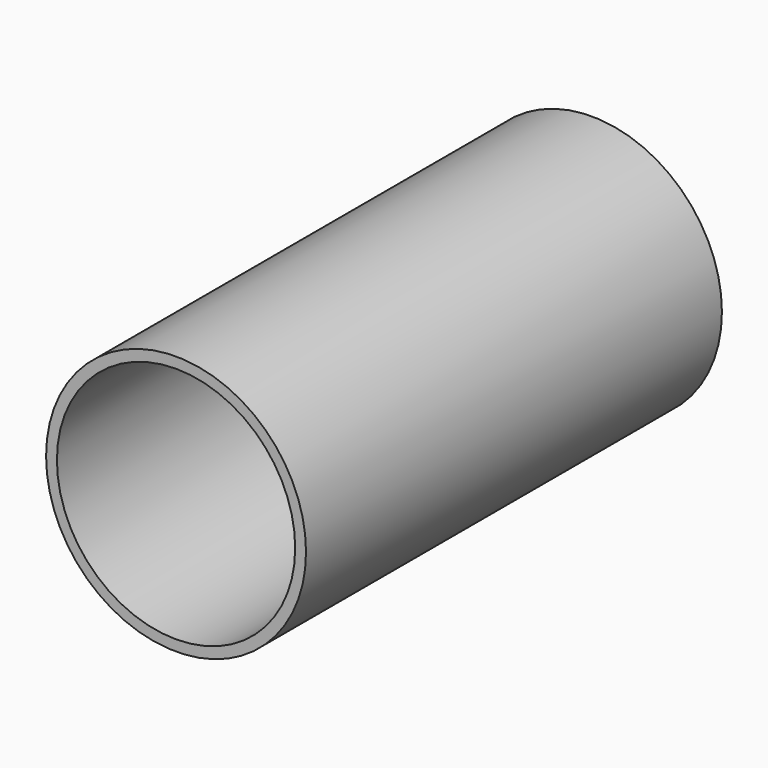
from build123d import *

# Parameters (mm, degrees)
F1_R     = 76.2
F2_DEPTH = 304.8
F3_T     = -6.35


# Not quite as in the source:
# - a variable given as a bare number and used for a length is read in inches; the dataset says mm whatever the document's units were


with BuildPart() as f2:
    # F1 (on Front) → F2 (new body)
    with BuildSketch(Plane.XZ):
        Circle(F1_R)
    extrude(amount=-F2_DEPTH)

    # F3
    f3_openings = [f2.faces().sort_by_distance(p)[0] for p in [
        (0, 0, 0),
        (0, 304.8, 0),
    ]]
    offset(amount=F3_T, openings=f3_openings)


solid = f2.part
